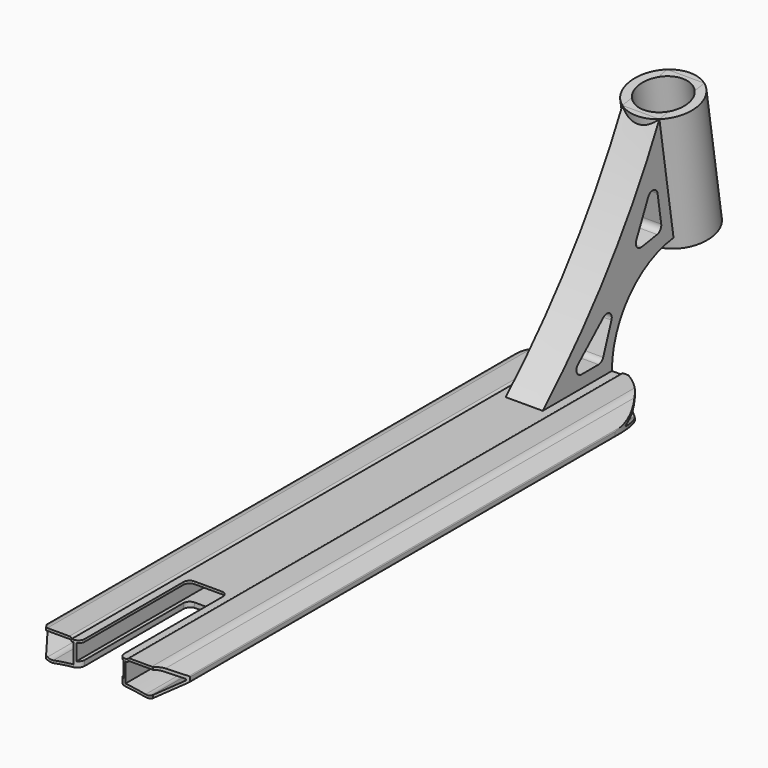
from build123d import *

# Parameters (mm, degrees)
F1_DEPTH       = 250
F2_W           = 38
F2_H           = 13
F3_DEPTH       = 250
F4_T1_DEPTH    = 509.3674969976
F5_R           = 9
F6_R           = 1
F8_DEPTH       = 500.001
F10_DEPTH      = 25
F11_DEPTH      = 22.2193051812
F11_DEPTH_BACK = 25.0010001
F13_DEPTH      = 22.219305294
F13_DEPTH_BACK = 1.3010001
F14_R          = 4.99999
F16_DEPTH      = 15
F17_R          = 27.4590604355
F18_DEPTH      = 100
F20_D          = 40
F22_DEPTH      = 72.5010001
F23_R          = 5


# Not quite as in the source:
# - a fillet or chamfer that OpenCascade refuses, or shapes differently, is made with other operations: its cross-section is extruded or revolved along the edge and cut away or added
# - a fillet or chamfer is up to 0.001 mm smaller than in the source, because OpenCascade refuses the exact size


with BuildPart() as f1:
    # F0 (on Front) → F1 (new body, symmetric)
    with BuildSketch(Plane.XZ):
        with BuildLine():
            Line((22.5, 0), (0, 0))
            Line((0, 0), (-22.5, 0))
            Line((-22.5, 0), (-22.5, 1.3))
            Line((-22.5, 1.3), (-45.5824640741, 1.3))
            Line((-45.5824640741, 1.3), (-57.5, -8.7))
            Line((-57.5, -8.7), (-57.5, -12.7))
            Line((-57.5, -12.7), (-40.1794919243, -22.7))
            ThreePointArc((-40.1794919243, -22.7), (0, -18.6224551416), (40.1794919243, -22.7))
            Line((40.1794919243, -22.7), (57.5, -12.7))
            Line((57.5, -12.7), (57.5, -8.7))
            Line((57.5, -8.7), (45.5824640741, 1.3))
            Line((45.5824640741, 1.3), (22.5, 1.3))
            Line((22.5, 1.3), (22.5, 0))
        make_face()
    extrude(amount=F1_DEPTH, both=True)

    # F2 (on Front) → F3 (cut, symmetric)
    with BuildSketch(Plane.XZ):
        with Locations((0, -8.5)):
            Rectangle(F2_W, F2_H)
    extrude(amount=F3_DEPTH, both=True, mode=Mode.SUBTRACT)

    # F4: fillet of radius 2 on 2 edges, made by hand

    # F4_s2 → F4_t1 (cut)
    with BuildSketch(Plane.XZ.offset(-254.6837484988)):
        with BuildLine():
            ThreePointArc((-24.3734993995, 1.3), (-23.2333239744, 0.9431676725), (-22.5, 0))
            Line((-22.5, 0), (-22.5, 1.3))
            Line((-22.5, 1.3), (-24.3734993995, 1.3))
        make_face()
        with BuildLine():
            ThreePointArc((24.3734993995, 1.3), (23.2333239744, 0.9431676725), (22.5, 0))
            Line((22.5, 0), (22.5, 1.3))
            Line((22.5, 1.3), (24.3734993995, 1.3))
        make_face()
    extrude(amount=F4_T1_DEPTH, mode=Mode.SUBTRACT)

    # F5
    f5_edges = [f1.edges().sort_by_distance(p)[0] for p in [
        (45.582464, 0, 1.3),
        (40.179492, 0, -22.7),
        (-45.582464, 0, 1.3),
        (-40.179492, 0, -22.7),
    ]]
    fillet(f5_edges, radius=F5_R)

    # F6
    f6_edges = [f1.edges().sort_by_distance(p)[0] for p in [
        (57.5, 0, -8.7),
        (57.5, 0, -12.7),
        (-57.5, 0, -8.7),
        (-57.5, 0, -12.7),
    ]]
    fillet(f6_edges, radius=F6_R)

    # F7 (on face) → F8 (cut, through all)
    with BuildSketch(Plane.XZ.offset(250)):
        with BuildLine():
            Line((21, -2), (21, -17.7170047426))
            ThreePointArc((21, -17.7170047426), (29.1789785809, -18.7410222645), (37.3093701274, -20.0978700124))
            ThreePointArc((37.3093701274, -20.0978700124), (39.7790673433, -20.1186780608), (42.1022690923, -19.2804830077))
            Line((42.1022690923, -19.2804830077), (55.6135241478, -11.4797562644))
            ThreePointArc((55.6135241478, -11.4797562644), (56.1097188459, -10.7008866033), (55.7563117574, -9.8476864174))
            Line((55.7563117574, -9.8476864174), (46.8062452335, -2.3376888982))
            ThreePointArc((46.8062452335, -2.3376888982), (44.7008729689, -1.1221516545), (42.3067319657, -0.7))
            Line((42.3067319657, -0.7), (24.3734993995, -0.7))
            ThreePointArc((24.3734993995, -0.7), (23.2333239744, -1.0568323275), (22.5, -2))
            Line((22.5, -2), (21, -2))
        make_face()
        with BuildLine():
            ThreePointArc((-42.1022690923, -19.2804830077), (-39.7790673433, -20.1186780608), (-37.3093701274, -20.0978700124))
            ThreePointArc((-37.3093701274, -20.0978700124), (-29.1789785809, -18.7410222645), (-21, -17.7170047426))
            Line((-21, -17.7170047426), (-21, -2))
            Line((-21, -2), (-22.5, -2))
            ThreePointArc((-22.5, -2), (-23.2333239744, -1.0568323275), (-24.3734993995, -0.7))
            Line((-24.3734993995, -0.7), (-42.3067319657, -0.7))
            ThreePointArc((-42.3067319657, -0.7), (-44.7008729689, -1.1221516545), (-46.8062452335, -2.3376888982))
            Line((-46.8062452335, -2.3376888982), (-55.7563117574, -9.8476864174))
            ThreePointArc((-55.7563117574, -9.8476864174), (-56.1097188459, -10.7008866033), (-55.6135241478, -11.4797562644))
            Line((-55.6135241478, -11.4797562644), (-42.1022690923, -19.2804830077))
        make_face()
    extrude(amount=-F8_DEPTH, mode=Mode.SUBTRACT)

    # F9 (on Top) → F10 (join)
    with BuildSketch(Plane.XY):
        with BuildLine():
            ThreePointArc((-57.5, 200), (0, 257.5), (57.5, 200))
            Line((57.5, 200), (57.5, 280))
            Line((57.5, 280), (-57.5, 280))
            Line((-57.5, 280), (-57.5, 200))
        make_face()
    extrude(amount=F10_DEPTH)

    # F9 (on Top) → F11 (cut, two sides)
    with BuildSketch(Plane.XY) as f11_sk:
        with BuildLine():
            ThreePointArc((-57.5, 200), (0, 257.5), (57.5, 200))
            Line((57.5, 200), (57.5, 280))
            Line((57.5, 280), (-57.5, 280))
            Line((-57.5, 280), (-57.5, 200))
        make_face()
    extrude(amount=-F11_DEPTH, mode=Mode.SUBTRACT)
    extrude(f11_sk.sketch, amount=F11_DEPTH_BACK, mode=Mode.SUBTRACT)

    # F12 (on Top) → F13 (cut, two sides)
    with BuildSketch(Plane.XY) as f13_sk:
        Polygon((-43.2975540478, -250), (-68, -216), (-68, -346), (68, -346), (68, -216), (43.2975540478, -250), (16, -250), (16, -140), (-16, -140), (-16, -250), align=None)
    extrude(amount=-F13_DEPTH, mode=Mode.SUBTRACT)
    extrude(f13_sk.sketch, amount=F13_DEPTH_BACK, mode=Mode.SUBTRACT)

    # F14 (radius 5 in the source; OpenCascade refuses exactly that, so slightly less here)
    f14_edges = [f1.edges().sort_by_distance(p)[0] for p in [
        (-16, -140, -17.131741),
        (-16, -140, -1),
        (16, -140, -17.131741),
        (16, -140, -1),
        (16, -250, -1),
        (-16, -250, -1),
    ]]
    fillet(f14_edges, radius=F14_R)

    # F15 (on Right) → F16 (join, symmetric)
    with BuildSketch(Plane.YZ):
        with BuildLine():
            ThreePointArc((298.1000497807, 160), (246.3415841777, 74.6179155324), (180, 0))
            Line((180, 0), (250, 0))
            ThreePointArc((250, 0), (267.8914074394, 46.7407165259), (312.4198451815, 69.5883700982))
            Line((312.4198451815, 69.5883700982), (313.7434962847, 61.2311659405))
            Line((313.7434962847, 61.2311659405), (359.1771599521, 68.4271513323))
            Line((359.1771599521, 68.4271513323), (343.5337134481, 167.1959853919))
            Line((343.5337134481, 167.1959853919), (298.1000497807, 160))
        make_face()
    extrude(amount=F16_DEPTH, both=True)

    # F17 (on face) → F18 (join, through all)
    with BuildSketch(Plane(origin=(0, -17.4263320856, 110.0255306005), x_dir=(1, 0, 0), z_dir=(0, -0.156434465, 0.9876883406))):
        with Locations((0, 342.4594579056)):
            Circle(F17_R)
    extrude(amount=-F18_DEPTH)

    # F20 (through all)
    with Locations(Plane(origin=(0, -17.4263320856, 110.0255306005), x_dir=(1, 0, 0), z_dir=(0, -0.156434465, 0.9876883406))):
        with Locations((0, 342.4594579056)):
            Hole(F20_D / 2)

    # F21 (on face) → F22 (cut, through all)
    with BuildSketch(Plane.YZ.offset(15)):
        Polygon((240, 10), (256.378660542, 55), (206, 10), align=None)
        Polygon((300.737923578, 79.4205881019), (293.6983726512, 123.8665634287), (270.737923578, 74.6690548922), align=None)
    extrude(amount=-F22_DEPTH, mode=Mode.SUBTRACT)

    # F23
    f23_edges = [f1.edges().sort_by_distance(p)[0] for p in [
        (0, 240, 10),
        (0, 300.737924, 79.420588),
        (0, 293.698373, 123.866563),
        (0, 270.737924, 74.669055),
        (0, 206, 10),
        (0, 256.378661, 55),
    ]]
    fillet(f23_edges, radius=F23_R)


solid = f1.part
